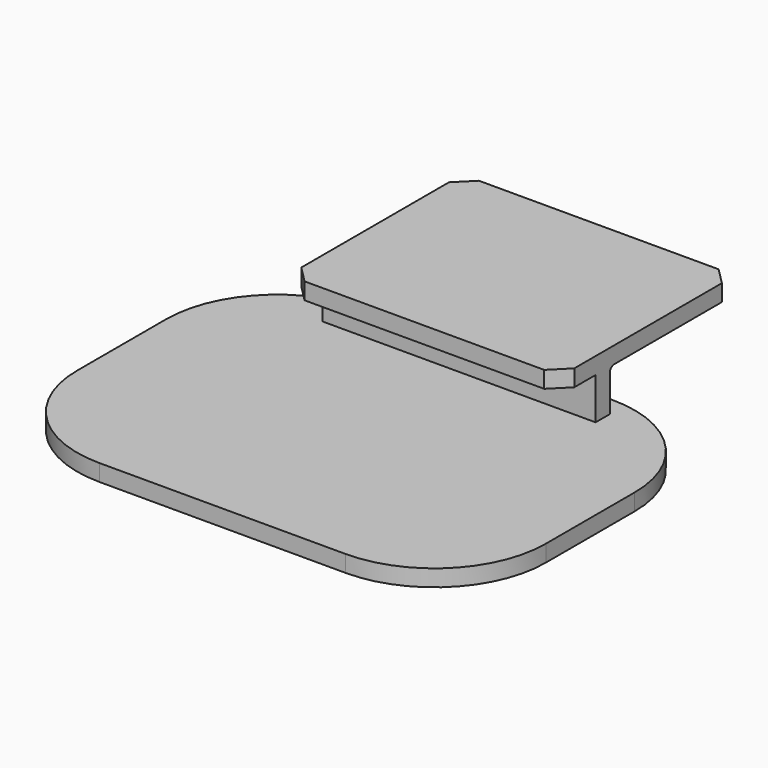
from build123d import *

# Parameters (mm, degrees)
F1_DEPTH      = 3
F2_W          = 49.1
F2_H          = 3.2
F3_DEPTH      = 13.5
F5_W          = 49.1
F5_H          = 39.2
F6_DEPTH      = 3
F7_SIZE       = 3
F8_SIZE       = 3
F9_SIZE       = 3
F10_SIZE      = 3
F11_R         = 1
F13_TEXT_SIZE = 9.581698955
F14_DEPTH     = 1


# Not quite as in the source:
# - Text() gives the source's letters only with a copy of the font that has no kerning and outlines rounded to 1/6400 em; it was checked with that copy


with BuildPart() as f1:
    # F0 (on Top) → F1 (new body)
    with BuildSketch(Plane.XY):
        with BuildLine():
            Line((22.15, 42.15), (-22.15, 42.15))
            ThreePointArc((-22.15, 42.15), (-36.2921356237, 36.2921356237), (-42.15, 22.15))
            Line((-42.15, 22.15), (-42.15, 2.15))
            ThreePointArc((-42.15, 2.15), (-36.2921356237, -11.9921356237), (-22.15, -17.85))
            Line((-22.15, -17.85), (22.15, -17.85))
            ThreePointArc((22.15, -17.85), (36.2921356237, -11.9921356237), (42.15, 2.15))
            Line((42.15, 2.15), (42.15, 22.15))
            ThreePointArc((42.15, 22.15), (36.2921356237, 36.2921356237), (22.15, 42.15))
        make_face()
    extrude(amount=F1_DEPTH)

    # F2 (on Top) → F3 (join)
    with BuildSketch(Plane.XY):
        with Locations((0, 36.95)):
            Rectangle(F2_W, F2_H)
    extrude(amount=F3_DEPTH)

    # F5 (on offset) → F6 (join)
    with BuildSketch(Plane.XY.offset(13.5)):
        with Locations((0, 47.15)):
            Rectangle(F5_W, F5_H)
    extrude(amount=-F6_DEPTH)

    # F7
    f7_edges = [f1.edges().sort_by_distance(p)[0] for p in [
        (24.55, 66.75, 12),
    ]]
    chamfer(f7_edges, length=F7_SIZE)

    # F8
    f8_edges = [f1.edges().sort_by_distance(p)[0] for p in [
        (-24.55, 66.75, 12),
    ]]
    chamfer(f8_edges, length=F8_SIZE)

    # F9
    f9_edges = [f1.edges().sort_by_distance(p)[0] for p in [
        (-24.55, 27.55, 12),
    ]]
    chamfer(f9_edges, length=F9_SIZE)

    # F10
    f10_edges = [f1.edges().sort_by_distance(p)[0] for p in [
        (24.55, 27.55, 12),
    ]]
    chamfer(f10_edges, length=F10_SIZE)

    # F11
    f11_edges = [f1.edges().sort_by_distance(p)[0] for p in [
        (0, 38.55, 10.5),
    ]]
    fillet(f11_edges, radius=F11_R)

    # F13 (on offset) → F14 (cut)
    with BuildSketch(Plane(origin=(0, 0, 0), x_dir=(1, 0, 0), z_dir=(0, 0, -1))):
        with Locations(Location((32.15, 7.85), (0, 0, 180))):
            Text('AB Designs', F13_TEXT_SIZE, font='Open Sans', text_align=(TextAlign.LEFT, TextAlign.BOTTOM))
    extrude(amount=-F14_DEPTH, mode=Mode.SUBTRACT)


solid = f1.part
